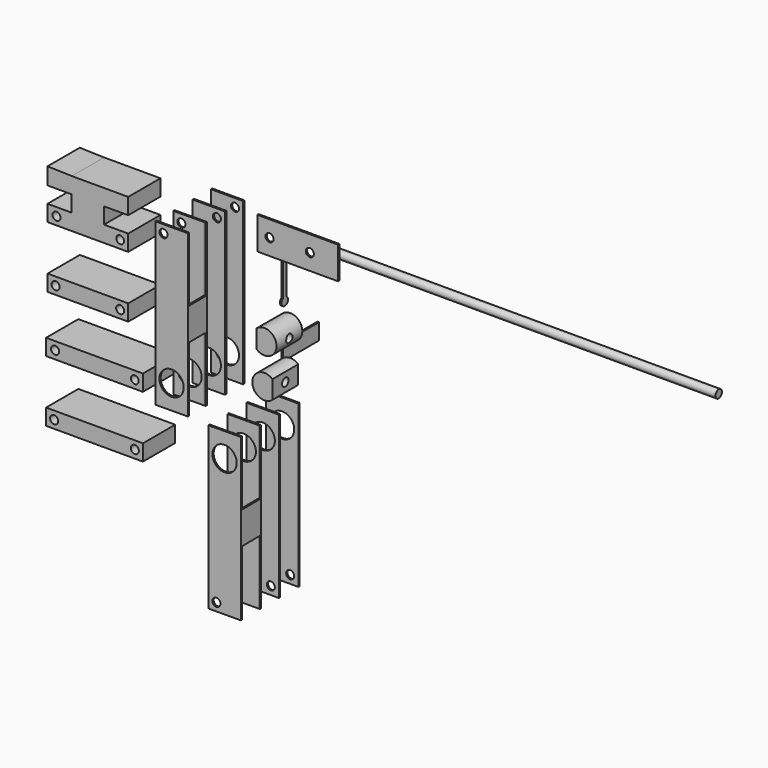
from build123d import *

# Parameters (mm, degrees)
F1_DEPTH  = 100
F2_R      = 7.5
F2_R_2    = 2.5
F3_DEPTH  = 15.001
F4_W      = 13
F4_H      = 40
F5_DEPTH  = 20.1627097718
F6_DEPTH  = 100
F7_R      = 7.5
F7_R_2    = 2.5
F8_DEPTH  = 16.001
F9_W      = 14
F9_H      = 40
F10_DEPTH = 20.1691592966
F11_W     = 50
F11_H     = 20
F11_R     = 2.5
F12_DEPTH = 1
F13_R     = 2.5
F13_R_2   = 7.5
F14_DEPTH = 45.1330833913
F15_R     = 7.5
F15_R_2   = 2.5
F16_DEPTH = 46.1330833913
F17_W     = 14
F17_H     = 40
F18_DEPTH = 53.5847666336
F19_W     = 13
F19_H     = 40
F20_DEPTH = 25
F22_DEPTH = 20
F23_R     = 2.5
F24_DEPTH = 250
F25_W     = 50
F25_H     = 10
F25_R     = 2.5
F26_DEPTH = 25
F25_R_2   = 2.4144593705
F25_W_2   = 60
F27_DEPTH = 25
F28_R     = 2.5
F29_DEPTH = 136.2251037518
F30_R     = 2.5
F31_DEPTH = 214.5146418358
F33_DEPTH = 1
F34_W     = 1
F34_H     = 10
F35_DEPTH = 25


# Not quite as in the source:
# - a feature names something its author has since deleted; it is built from what else it names


with BuildPart() as f1:
    # F0 (on Top) → F1 (new body)
    with BuildSketch(Plane.XY):
        Polygon((0, 14), (0, 15), (-20, 15), (-20, 0), (0, 0), (0, 1), (-19, 1), (-19, 14), align=None)
    extrude(amount=F1_DEPTH)

    # F2 (on face) → F3 (cut, through all)
    with BuildSketch(Plane.XZ):
        with Locations((-10, 15)):
            Circle(F2_R)
        with Locations((-5, 95)):
            Circle(F2_R_2)
    extrude(amount=-F3_DEPTH, mode=Mode.SUBTRACT)

    # F4 (on face) → F5 (cut, through all)
    with BuildSketch(Plane(origin=(-20, 0, 0), x_dir=(0, -1, 0), z_dir=(-1, 0, 0))):
        with Locations((-7.5, 20)):
            Rectangle(F4_W, F4_H)
        with Locations((-7.5, 80)):
            Rectangle(F4_W, F4_H)
    extrude(amount=-F5_DEPTH, mode=Mode.SUBTRACT)


with BuildPart() as f1b:
    # F0 (on Top) → F1, piece 2 (new body)
    with BuildSketch(Plane.XY):
        Polygon((0.051417134, -13.985459061), (-19.9480422158, -14.1325159114), (-19.9406893732, -15.1324888789), (-0.941202991, -14.992784871), (-0.8456160382, -27.9924334484), (-19.837749578, -28.1320833905), (-19.837749578, -29.1321104238), (0.1617097718, -28.9850535734), align=None)
    extrude(amount=F1_DEPTH)

    # F13 (on face) → F14 (cut, through all)
    with BuildSketch(Plane(origin=(0.2131255159, -28.9846755113, 0), x_dir=(0.9999729675, 0.0073528425, 0), z_dir=(0.0073528425, -0.9999729675, 0))):
        with Locations((-15.051417134, 95)):
            Circle(F13_R)
        with Locations((-10.051417134, 15)):
            Circle(F13_R_2)
    extrude(amount=-F14_DEPTH, mode=Mode.SUBTRACT)

    # F19 (on face) → F20 (cut)
    with BuildSketch(Plane(origin=(-0.0514157441, -0.0003780621, 0), x_dir=(-0.0073528425, 0.9999729675, 0), z_dir=(0.9999729675, 0.0073528425, 0))):
        with Locations((-21.485459061, 20)):
            Rectangle(F19_W, F19_H)
        with Locations((-21.485459061, 80)):
            Rectangle(F19_W, F19_H)
    extrude(amount=-F20_DEPTH, mode=Mode.SUBTRACT)


with BuildPart() as f6:
    # F0 (on Top) → F6 (new body)
    with BuildSketch(Plane.XY):
        Polygon((33.4159745649, 0), (33.4159745649, 1), (14.4159745649, 1), (14.4159745649, 15), (33.4159745649, 15), (33.4159745649, 16), (13.4159745649, 16), (13.4159745649, 0), align=None)
    extrude(amount=-F6_DEPTH)

    # F7 (on face) → F8 (cut, through all)
    with BuildSketch(Plane.XZ):
        with Locations((23.4159745649, -15)):
            Circle(F7_R)
        with Locations((28.4159745649, -95)):
            Circle(F7_R_2)
    extrude(amount=-F8_DEPTH, mode=Mode.SUBTRACT)

    # F9 (on face) → F10 (cut, through all)
    with BuildSketch(Plane(origin=(13.4159745649, 0, 0), x_dir=(0, -1, 0), z_dir=(-1, 0, 0))):
        with Locations((-8, -20)):
            Rectangle(F9_W, F9_H)
        with Locations((-8, -80)):
            Rectangle(F9_W, F9_H)
    extrude(amount=-F10_DEPTH, mode=Mode.SUBTRACT)


with BuildPart() as f6b:
    # F0 (on Top) → F6, piece 2 (new body)
    with BuildSketch(Plane.XY):
        Polygon((33.4664883811, -13.7397566624), (13.4670290313, -13.8868135128), (13.4743818739, -14.8867864803), (32.4738682561, -14.7470824724), (32.5768080514, -28.7467040172), (13.5846745117, -28.8863539594), (13.5846745117, -29.8863809926), (33.5841338614, -29.7393241422), align=None)
    extrude(amount=-F6_DEPTH)

    # F15 (on face) → F16 (cut, through all)
    with BuildSketch(Plane(origin=(0.2204783584, -29.9846484788, 0), x_dir=(0.9999729675, 0.0073528425, 0), z_dir=(0.0073528425, -0.9999729675, 0))):
        with Locations((23.3645574309, -15)):
            Circle(F15_R)
        with Locations((18.3645574309, -95)):
            Circle(F15_R_2)
    extrude(amount=-F16_DEPTH, mode=Mode.SUBTRACT)

    # F17 (on face) → F18 (cut, through all)
    with BuildSketch(Plane(origin=(33.3636555031, 0.2453243365, 0), x_dir=(-0.0073528425, 0.9999729675, 0), z_dir=(0.9999729675, 0.0073528425, 0))):
        with Locations((-21.985459061, -20)):
            Rectangle(F17_W, F17_H)
        with Locations((-21.985459061, -80)):
            Rectangle(F17_W, F17_H)
    extrude(amount=-F18_DEPTH, mode=Mode.SUBTRACT)


with BuildPart() as f12:
    # F11 (on Front) → F12 (new body)
    with BuildSketch(Plane.XZ):
        with Locations((45.8931141218, 95.3558683395)):
            Rectangle(F11_W, F11_H)
        with Locations((28.3931141218, 95.3558683395)):
            Circle(F11_R, mode=Mode.SUBTRACT)
        with Locations((53.3931141218, 95.3558683395)):
            Circle(F11_R, mode=Mode.SUBTRACT)
    extrude(amount=F12_DEPTH)


with BuildPart() as f22:
    # F21 (on Front) → F22 (new body)
    with BuildSketch(Plane.XZ):
        with BuildLine():
            Line((35.4863581642, 55.8813297105), (35.4863581642, 44.6073331245))
            ThreePointArc((35.4863581642, 44.6073331245), (47.9335038306, 50.2443314175), (35.4863581642, 55.8813297105))
        make_face()
    extrude(amount=F22_DEPTH)

    # F30 (on face) → F31 (cut, through all)
    with BuildSketch(Plane(origin=(35.4863581642, 0, 0), x_dir=(0, -1, 0), z_dir=(-1, 0, 0))):
        with Locations((10, 50.2443314175)):
            Circle(F30_R)
    extrude(amount=-F31_DEPTH, mode=Mode.SUBTRACT)


with BuildPart() as f22b:
    # F21 (on Front) → F22, piece 2 (new body)
    with BuildSketch(Plane.XZ):
        with BuildLine():
            Line((45.380649497, 20.1312099156), (45.380649497, 31.4052065016))
            ThreePointArc((45.380649497, 31.4052065016), (32.9335038306, 25.7682082086), (45.380649497, 20.1312099156))
        make_face()
    extrude(amount=F22_DEPTH)

    # F28 (on face) → F29 (cut, through all)
    with BuildSketch(Plane.YZ.offset(45.380649497)):
        with Locations((-10, 25.7682082086)):
            Circle(F28_R)
    extrude(amount=-F29_DEPTH, mode=Mode.SUBTRACT)


with BuildPart() as f24:
    # F23 (on Right) → F24 (new body)
    with BuildSketch(Plane.YZ):
        with Locations((69.883659482, 53.4276850522)):
            Circle(F23_R)
    extrude(amount=F24_DEPTH)


with BuildPart() as f26:
    # F25 (on Front) → F26 (new body)
    with BuildSketch(Plane.XZ):
        with Locations((-64.9493469292, 42.0624911785)):
            Rectangle(F25_W, F25_H)
        with Locations((-84.9493469292, 42.0624911785)):
            Circle(F25_R, mode=Mode.SUBTRACT)
        with Locations((-44.9493469292, 42.0624911785)):
            Circle(F25_R, mode=Mode.SUBTRACT)
    extrude(amount=F26_DEPTH)


with BuildPart() as f26b:
    # F25 (on Front) → F26, piece 2 (new body)
    with BuildSketch(Plane.XZ):
        Polygon((-89.9493469292, 85.124527216), (-89.9493469292, 75.124527216), (-39.9493469292, 75.124527216), (-39.9493469292, 85.124527216), (-54.9493469292, 85.124527216), (-54.9493469292, 95.124527216), (-39.9493469292, 95.124527216), (-39.9493469292, 105.124527216), (-54.9493469292, 105.124527216), (-64.9493469292, 105.124527216), (-74.9493469292, 105.124527216), (-89.9493469292, 105.5638343096), (-89.9493469292, 95.124527216), (-74.9493469292, 95.124527216), (-74.9493469292, 85.124527216), align=None)
        with Locations((-84.3778774142, 80.124527216)):
            Circle(F25_R, mode=Mode.SUBTRACT)
        with Locations((-44.9493469292, 80.124527216)):
            Circle(F25_R_2, mode=Mode.SUBTRACT)
    extrude(amount=F26_DEPTH)


with BuildPart() as f27:
    # F25 (on Front) → F27 (new body)
    with BuildSketch(Plane.XZ):
        with Locations((-60.8434542548, -31.3186603598)):
            Rectangle(F25_W_2, F25_H)
        with Locations((-85.8434542548, -31.3186603598)):
            Circle(F25_R, mode=Mode.SUBTRACT)
        with Locations((-35.8434542548, -31.3186603598)):
            Circle(F25_R, mode=Mode.SUBTRACT)
    extrude(amount=F27_DEPTH)


with BuildPart() as f27b:
    # F25 (on Front) → F27, piece 2 (new body)
    with BuildSketch(Plane.XZ):
        with Locations((-60.8434542548, 6.7433756776)):
            Rectangle(F25_W_2, F25_H)
        with Locations((-85.2719847398, 6.7433756776)):
            Circle(F25_R, mode=Mode.SUBTRACT)
        with Locations((-35.8434542548, 6.7433756776)):
            Circle(F25_R_2, mode=Mode.SUBTRACT)
    extrude(amount=F27_DEPTH)


with BuildPart() as f33:
    # F32 (on Right) → F33 (new body)
    with BuildSketch(Plane.YZ):
        with BuildLine():
            Line((47.762863338, 8.6800148711), (47.762863338, 20.4667558931))
            ThreePointArc((47.762863338, 20.4667558931), (46.3052242994, 24.9978365004), (44.8475852609, 20.4667558931))
            Line((44.8475852609, 20.4667558931), (44.8475852609, 8.6800148711))
            Line((44.8475852609, 8.6800148711), (44.8475852609, 0))
            Line((44.8475852609, 0), (47.762863338, 0))
            Line((47.762863338, 0), (47.762863338, 8.6800148711))
        make_face()
    extrude(amount=-F33_DEPTH)

    # F34 (on face) → F35 (join)
    with BuildSketch(Plane(origin=(0, 47.762863338, 0), x_dir=(-1, 0, 0), z_dir=(0, 1, 0))):
        with Locations((0.5, 5)):
            Rectangle(F34_W, F34_H)
    extrude(amount=F35_DEPTH)


with BuildPart() as f33b:
    # F32 (on Right) → F33, piece 2 (new body)
    with BuildSketch(Plane.YZ):
        with BuildLine():
            ThreePointArc((44.8475852609, 34.1576339639), (46.3052242994, 29.6265533566), (47.762863338, 34.1576339639))
            Line((47.762863338, 34.1576339639), (47.762863338, 45.944374986))
            Line((47.762863338, 45.944374986), (47.762863338, 54.6243898571))
            Line((47.762863338, 54.6243898571), (44.8475852609, 54.6243898571))
            Line((44.8475852609, 54.6243898571), (44.8475852609, 45.944374986))
            Line((44.8475852609, 45.944374986), (44.8475852609, 34.1576339639))
        make_face()
    extrude(amount=-F33_DEPTH)


solid = Compound([f1.part, f1b.part, f6.part, f6b.part, f12.part, f22.part, f22b.part, f24.part, f26.part, f26b.part, f27.part, f27b.part, f33.part, f33b.part])
